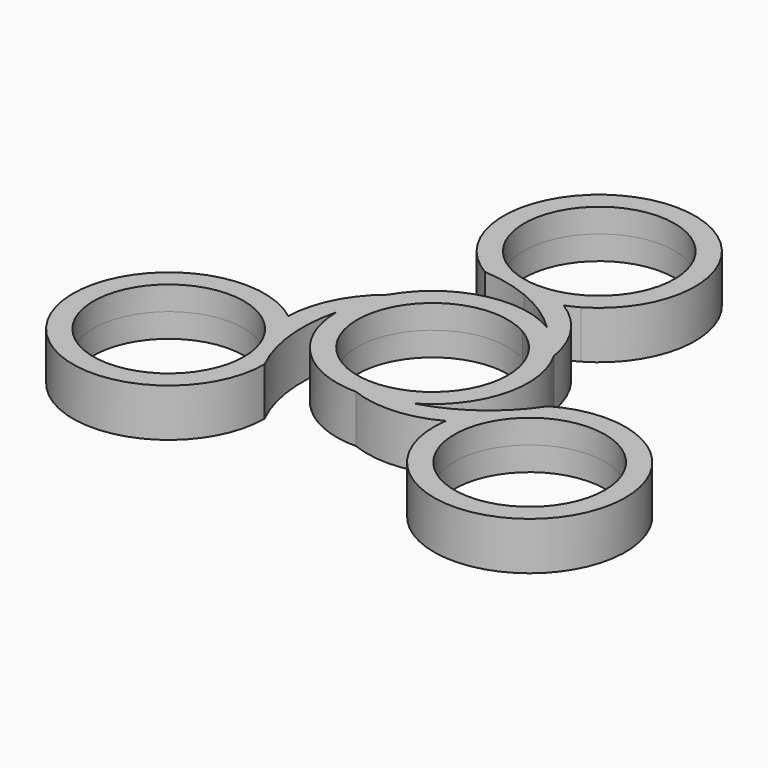
from build123d import *

# Parameters (mm, degrees)
F0_R     = 11
F1_DEPTH = 3.5


# Not quite as in the source:
# - a feature of the source that left no trace in its solid (it failed there, or was rolled back) is left out


with BuildPart() as f1:
    # F0 (on Top) → F1 (new body, symmetric)
    with BuildSketch(Plane.XY):
        with BuildLine():
            ThreePointArc((9.5262794416, 5.5), (10.6251840892, 2.8470094961), (11, 0))
            ThreePointArc((11, 0), (-9.5262794416, -5.5), (5.5, 9.5262794416))
            Line((5.5, 9.5262794416), (7, 12.124355653))
            ThreePointArc((7, 12.124355653), (-3.6234666314, 13.522961568), (-12.124355653, 7))
            ThreePointArc((-12.124355653, 7), (-13.522961568, 3.6234666314), (-14, 0))
            ThreePointArc((-14, 0), (-13.522961568, -3.6234666314), (-12.124355653, -7))
            ThreePointArc((-12.124355653, -7), (-9.8994949366, -9.8994949366), (-7, -12.124355653))
            ThreePointArc((-7, -12.124355653), (-3.6234666314, -13.522961568), (0, -14))
            ThreePointArc((0, -14), (3.6234666314, -13.522961568), (7, -12.124355653))
            ThreePointArc((7, -12.124355653), (13.522961568, -3.6234666314), (12.124355653, 7))
            Line((12.124355653, 7), (9.5262794416, 5.5))
        make_face()
        with BuildLine():
            ThreePointArc((5.5, 9.5262794416), (7.7781745931, 7.7781745931), (9.5262794416, 5.5))
            Line((9.5262794416, 5.5), (12.124355653, 7))
            ThreePointArc((12.124355653, 7), (9.7975961228, 12.9972967743), (5.1726973399, 17.4685035196))
            ThreePointArc((5.1726973399, 17.4685035196), (6.1042077739, 17.8616349143), (7, 18.3304848581))
            ThreePointArc((7, 18.3304848581), (0, 44.4548405111), (-7, 18.3304848581))
            ThreePointArc((-7, 18.3304848581), (-3.4339564303, 17.8173408021), (0, 16.7274202555))
            ThreePointArc((0, 16.7274202555), (3.7217872887, 14.7631656496), (7, 12.124355653))
            Line((7, 12.124355653), (5.5, 9.5262794416))
        make_face()
        with BuildLine():
            ThreePointArc((5.5, 20.9285610695), (2.8470094961, 19.8296564219), (0, 19.4548405111))
            ThreePointArc((0, 19.4548405111), (-2.8470094961, 19.8296564219), (-5.5, 20.9285610695))
            ThreePointArc((-5.5, 20.9285610695), (-5.5, 39.9811199527), (11, 30.4548405111))
            ThreePointArc((11, 30.4548405111), (9.5262794416, 24.9548405111), (5.5, 20.9285610695))
        make_face(mode=Mode.SUBTRACT)
        with BuildLine():
            ThreePointArc((-14, 0), (-13.522961568, 3.6234666314), (-12.124355653, 7))
            ThreePointArc((-12.124355653, 7), (-16.1547872485, 1.9863187512), (-17.714516484, -4.2545644573))
            ThreePointArc((-17.714516484, -4.2545644573), (-18.5207334759, -3.644418455), (-19.3746655508, -3.1030646026))
            ThreePointArc((-19.3746655508, -3.1030646026), (-38.4990212038, -22.2274202555), (-12.3746655508, -15.2274202555))
            ThreePointArc((-12.3746655508, -15.2274202555), (-14.5592658851, -7.760146629), (-14, 0))
        make_face()
        with Locations((-26.3746655508, -15.2274202555)):
            Circle(F0_R, mode=Mode.SUBTRACT)
        with BuildLine():
            ThreePointArc((19.3746655508, -3.1030646026), (14.0001170604, -8.7286208024), (7, -12.124355653))
            ThreePointArc((7, -12.124355653), (3.6234666314, -13.522961568), (0, -14))
            ThreePointArc((0, -14), (6.3571911257, -14.9836155256), (12.5418191441, -13.2139390623))
            ThreePointArc((12.5418191441, -13.2139390623), (12.416525702, -14.2172164593), (12.3746655508, -15.2274202555))
            ThreePointArc((12.3746655508, -15.2274202555), (38.4990212038, -22.2274202555), (19.3746655508, -3.1030646026))
        make_face()
        with Locations((26.3746655508, -15.2274202555)):
            Circle(F0_R, mode=Mode.SUBTRACT)
    extrude(amount=F1_DEPTH, both=True)


solid = f1.part
